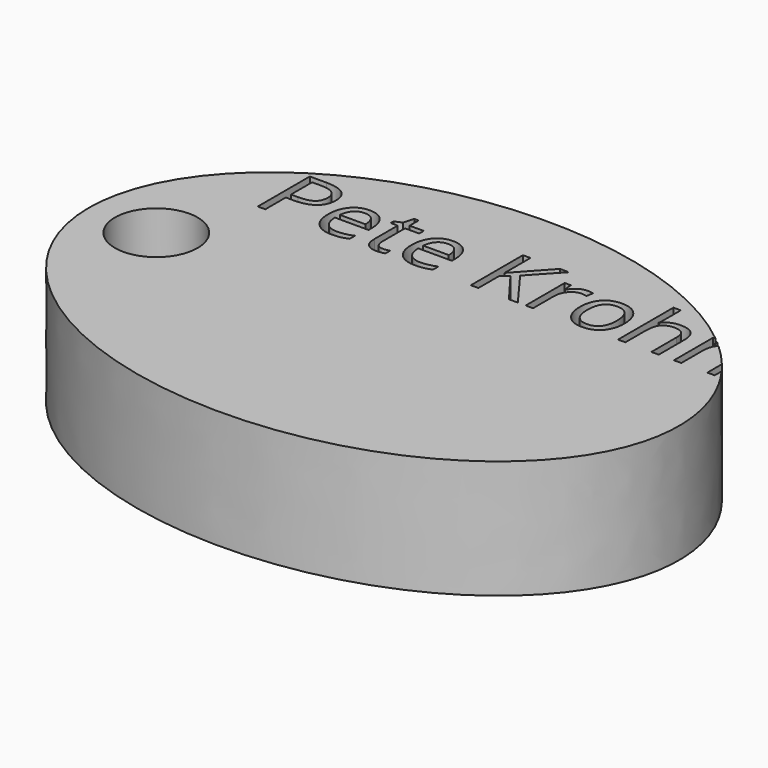
from build123d import *

# Parameters (mm, degrees)
F1_DEPTH     = 5.08
F2_R         = 1.7754574615
F3_DEPTH     = 7.62
F4_TEXT_SIZE = 3.9168502466
F5_DEPTH     = 2.54


# Not quite as in the source:
# - Text() gives the source's letters only with a copy of the font that has no kerning and outlines rounded to 1/6400 em; it was checked with that copy


with BuildPart() as f1:
    # F0 (on Top) → F1 (new body)
    with BuildSketch(Plane.XY):
        with BuildLine():
            add(Edge.make_bspline(
                [(-12.6803750172, 0), (-12.6803750172, -15.3074385485), (6.3401875086, -7.6537192743), (25.3607500345, 0), (6.3401875086, 7.6537192743), (-12.6803750172, 15.3074385485), (-12.6803750172, 0)],
                knots=[0, 0, 0, 2.0943951024, 2.0943951024, 4.1887902048, 4.1887902048, 6.2831853072, 6.2831853072, 6.2831853072], degree=2, weights=[1, 0.5, 1, 0.5, 1, 0.5, 1]))
        make_face()
    extrude(amount=F1_DEPTH)

    # F2 (on face) → F3 (cut)
    with BuildSketch(Plane.XY.offset(5.08)):
        with Locations((-9.7794607282, 0)):
            Circle(F2_R)
    extrude(amount=-F3_DEPTH, mode=Mode.SUBTRACT)

    # F4 (on face) → F5 (cut)
    with BuildSketch(Plane.XY.offset(5.08)):
        with Locations((-8.6965223771, 3.6116861475)):
            Text('Pete Krohn', F4_TEXT_SIZE, font='Open Sans', text_align=(TextAlign.LEFT, TextAlign.BOTTOM))
    extrude(amount=-F5_DEPTH, mode=Mode.SUBTRACT)


solid = f1.part
